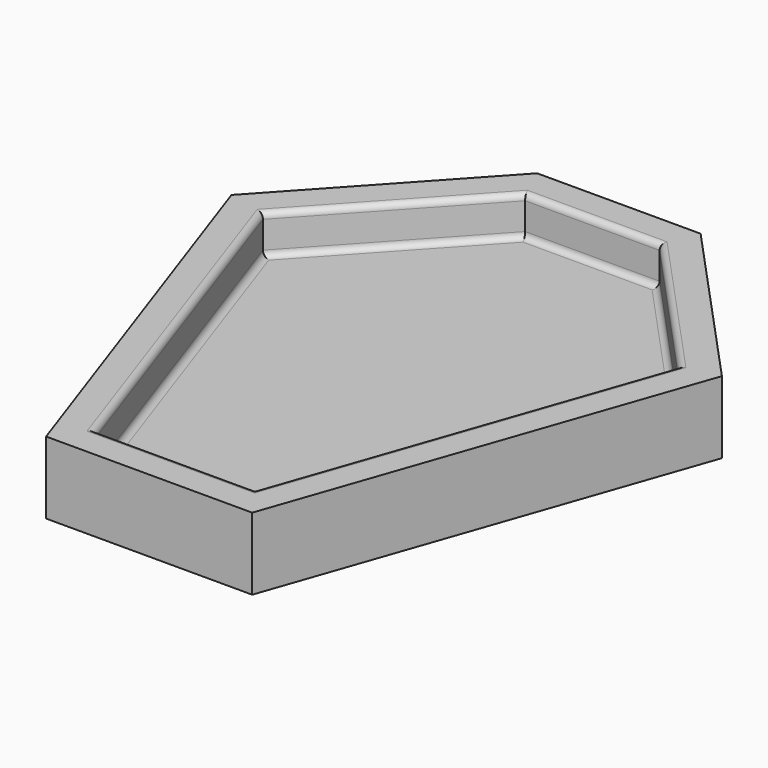
from build123d import *

# Parameters (mm, degrees)
F1_DEPTH = 304.8
F2_T     = -139.7
F3_R     = 25.4


# Not quite as in the source:
# - a feature of the source that left no trace in its solid (it failed there, or was rolled back) is left out


with BuildPart() as f1:
    # F0 (on Top) → F1 (new body)
    with BuildSketch(Plane.XY):
        Polygon((-434.9041368839, -1163.7434696012), (0, -1163.7434696012), (434.9041368839, -1163.7434696012), (1034.7719199285, 563.8757253794), (344.9239733095, 1313.7104347737), (0, 1313.7104347737), (-344.9239733095, 1313.7104347737), (-1034.7719199285, 563.8757253794), align=None)
    extrude(amount=F1_DEPTH)

    # F2
    f2_openings = [f1.faces().sort_by_distance(p)[0] for p in [
        (0, 124.086799, 304.8),
    ]]
    offset(amount=F2_T, openings=f2_openings)

    # F3
    f3_edges = [f1.edges().sort_by_distance(p)[0] for p in [
        (-579.508648, 852.392778, 304.8),
        (0, 1174.010435, 304.8),
        (579.508648, 852.392778, 304.8),
        (605.463112, -246.634174, 304.8),
        (0, -1024.04347, 304.8),
        (-605.463112, -246.634174, 304.8),
        (-605.463112, -246.634174, 139.7),
        (0, -1024.04347, 139.7),
        (605.463112, -246.634174, 139.7),
        (579.508648, 852.392778, 139.7),
        (0, 1174.010435, 139.7),
        (-579.508648, 852.392778, 139.7),
    ]]
    fillet(f3_edges, radius=F3_R)


solid = f1.part
